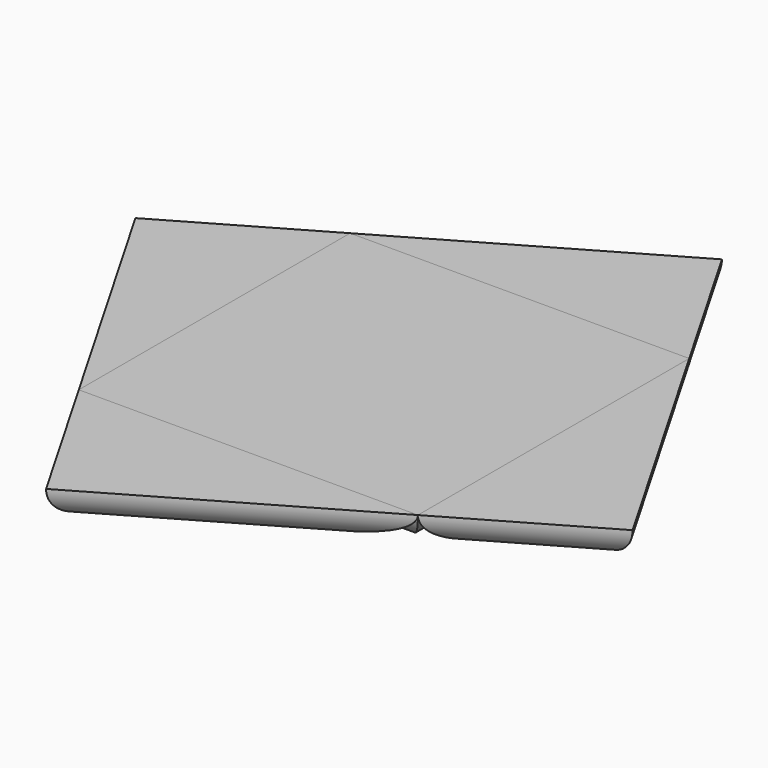
from build123d import *

# Parameters (mm, degrees)
F0_W     = 200
F0_H     = 200
F1_DEPTH = 18
F2_DEPTH = 18
F3_R     = 17.99999
F3_2_R   = 17.99999
F3_3_R   = 17.99999
F3_4_R   = 17.99999
F3_5_R   = 17.99999


# Not quite as in the source:
# - a fillet or chamfer is up to 0.001 mm smaller than in the source, because OpenCascade refuses the exact size


with BuildPart() as f1:
    # F0 (on Top) → F1 (new body)
    with BuildSketch(Plane.XY):
        Rectangle(F0_W, F0_H)
    extrude(amount=-F1_DEPTH)

    # F3 (radius 18 in the source; OpenCascade refuses exactly that, so slightly less here)
    f3_edges = [f1.edges().sort_by_distance(p)[0] for p in [
        (0, -100, -18),
        (100, 0, -18),
        (0, 100, -18),
        (-100, 0, -18),
    ]]
    fillet(f3_edges, radius=F3_R)


with BuildPart() as f2:
    # F0 (on Top) → F2 (new body)
    with BuildSketch(Plane.XY):
        Polygon((-186.6025403784, 50), (-100, -100), (-100, 100), align=None)
    extrude(amount=-F2_DEPTH)

    # F3#5 (radius 18 in the source; OpenCascade refuses exactly that, so slightly less here)
    f3_5_edges = [f2.edges().sort_by_distance(p)[0] for p in [
        (-100, 0, -18),
        (-143.30127, -25, -18),
        (-143.30127, 75, -18),
    ]]
    fillet(f3_5_edges, radius=F3_5_R)


with BuildPart() as f2b:
    # F0 (on Top) → F2, piece 2 (new body)
    with BuildSketch(Plane.XY):
        Polygon((-100, 100), (100, 100), (50, 186.6025403784), align=None)
    extrude(amount=-F2_DEPTH)

    # F3#4 (radius 18 in the source; OpenCascade refuses exactly that, so slightly less here)
    f3_4_edges = [f2b.edges().sort_by_distance(p)[0] for p in [
        (0, 100, -18),
        (-25, 143.30127, -18),
        (75, 143.30127, -18),
    ]]
    fillet(f3_4_edges, radius=F3_4_R)


with BuildPart() as f2c:
    # F0 (on Top) → F2, piece 3 (new body)
    with BuildSketch(Plane.XY):
        Polygon((100, 100), (100, -100), (186.6025403784, -50), align=None)
    extrude(amount=-F2_DEPTH)

    # F3#3 (radius 18 in the source; OpenCascade refuses exactly that, so slightly less here)
    f3_3_edges = [f2c.edges().sort_by_distance(p)[0] for p in [
        (100, 0, -18),
        (143.30127, 25, -18),
        (143.30127, -75, -18),
    ]]
    fillet(f3_3_edges, radius=F3_3_R)


with BuildPart() as f2d:
    # F0 (on Top) → F2, piece 4 (new body)
    with BuildSketch(Plane.XY):
        Polygon((-50, -186.6025403784), (100, -100), (-100, -100), align=None)
    extrude(amount=-F2_DEPTH)

    # F3#2 (radius 18 in the source; OpenCascade refuses exactly that, so slightly less here)
    f3_2_edges = [f2d.edges().sort_by_distance(p)[0] for p in [
        (0, -100, -18),
        (25, -143.30127, -18),
        (-75, -143.30127, -18),
    ]]
    fillet(f3_2_edges, radius=F3_2_R)


solid = Compound([f1.part, f2.part, f2b.part, f2c.part, f2d.part])
